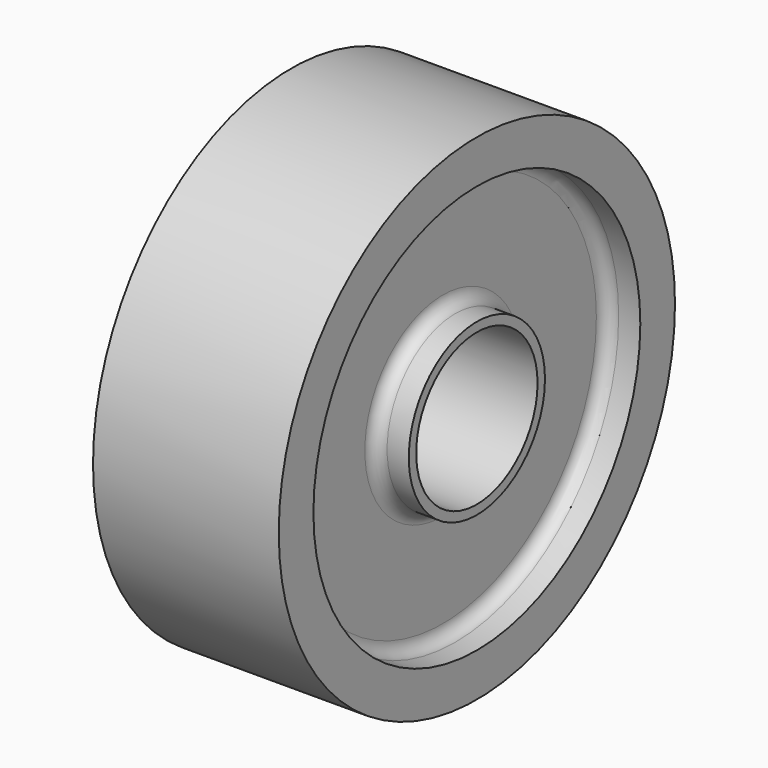
from build123d import *

# Parameters (mm, degrees)
F0_R          = 101.6
F0_R_2        = 83.82
F1_DEPTH      = 38.1
F1_DEPTH_BACK = 38.1
F0_R_3        = 34.925
F0_R_4        = 31.115
F2_DEPTH      = 24.13
F2_DEPTH_BACK = 24.13
F3_R          = 5.08


# Not quite as in the source:
# - a length typed as a fraction of an inch, garbled in the dataset ("3 / 203.2 mm" for 3/8 in), is restored


with BuildPart() as f1:
    # F0 (on Right) → F1 (new body, two sides)
    with BuildSketch(Plane.YZ) as f1_sk:
        Circle(F0_R)
        Circle(F0_R_2, mode=Mode.SUBTRACT)
    extrude(amount=F1_DEPTH)
    extrude(f1_sk.sketch, amount=-F1_DEPTH_BACK)



with BuildPart() as f1b:
    # F0 (on Right) → F1, piece 2 (new body, two sides)
    with BuildSketch(Plane.YZ) as f1_2_sk:
        Circle(F0_R_3)
        Circle(F0_R_4, mode=Mode.SUBTRACT)
    extrude(amount=F1_DEPTH)
    extrude(f1_2_sk.sketch, amount=-F1_DEPTH_BACK)


with BuildPart() as f1_1:
    add(f1.part)

    add(f1b.part)  # F2 merges F1b
    # F0 (on Right) → F2 (join, two sides)
    with BuildSketch(Plane.YZ) as f2_sk:
        Circle(F0_R_2)
        Circle(F0_R_3, mode=Mode.SUBTRACT)
    extrude(amount=F2_DEPTH)
    extrude(f2_sk.sketch, amount=-F2_DEPTH_BACK)

    # F3
    f3_edges = [f1_1.edges().sort_by_distance(p)[0] for p in [
        (24.13, -34.925, 0),
        (24.13, -83.82, 0),
        (-24.13, -34.925, 0),
        (-24.13, -83.82, 0),
    ]]
    fillet(f3_edges, radius=F3_R)


solid = f1_1.part
